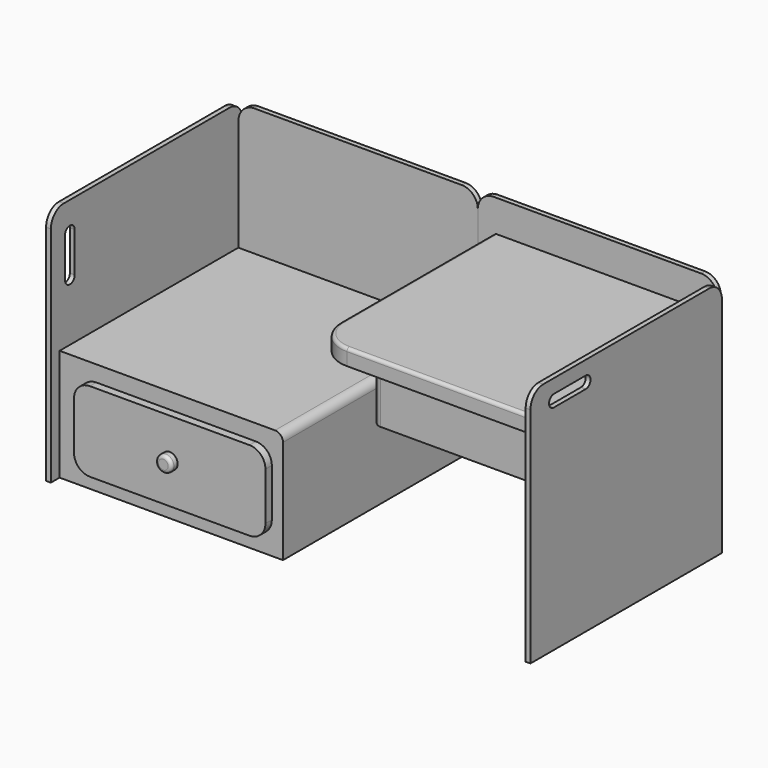
from build123d import *

# Parameters (mm, degrees)
F0_W      = 38.1
F0_H      = 38.1
F2_DEPTH  = 0.762
F1_W      = 38.1
F1_H      = 38.1
F3_DEPTH  = 0.762
F4_W      = 35.56
F4_H      = 35.56
F5_DEPTH  = 17.78
F8_W      = 30.48
F8_H      = 30.48
F9_DEPTH  = 10.16
F7_W      = 35.56
F7_H      = 35.56
F10_DEPTH = 2.54
F11_W     = 30.48
F11_H     = 12.7
F12_DEPTH = 1.27
F13_R     = 1.27
F14_DEPTH = 1.27
F16_R     = 1.27
F17_DEPTH = 2.54
F15_W     = 25.4
F15_H     = 7.62
F18_DEPTH = 1.27
F19_R     = 2.54
F19_2_R   = 2.54
F19_3_R   = 2.54
F20_R     = 5.08
F21_R     = 1.27
F21_2_R   = 1.27
F23_DEPTH = 12.7
F24_DEPTH = 0.762
F26_W     = 38.1
F26_H     = 38.1
F27_DEPTH = 0.762
F29_DEPTH = 12.7
F30_R     = 2.54
F30_2_R   = 2.54
F31_T     = 1.27
F33_DEPTH = 25.4
F34_R     = 0.508
F35_R     = 0.508
F36_R     = 0.508
F38_R     = 1.27


# Not quite as in the source:
# - two fillets or chamfers of one size are made in one step
# - a shell that OpenCascade refuses in one call is made with other operations: the cavity is built on its own and cut out
# - a feature names something its author has since deleted; it is built from what else it names


with BuildPart() as f2:
    # F0 (on Right) → F2 (new body)
    with BuildSketch(Plane.YZ):
        with Locations((-19.05, 19.05)):
            Rectangle(F0_W, F0_H)
    extrude(amount=-F2_DEPTH)

    # F19
    f19_edges = [f2.edges().sort_by_distance(p)[0] for p in [
        (-0.381, -38.1, 38.1),
        (-0.381, 0, 38.1),
    ]]
    fillet(f19_edges, radius=F19_R)

    # F22 (on face) → F23 (cut)
    with BuildSketch(Plane.YZ):
        with BuildLine():
            ThreePointArc((35.283215344, 34.4806989491), (34.330715344, 35.4331989491), (33.378215344, 34.4806989491))
            Line((33.378215344, 34.4806989491), (33.378215344, 28.1306989491))
            ThreePointArc((33.378215344, 28.1306989491), (34.330715344, 27.1781989491), (35.283215344, 28.1306989491))
            Line((35.283215344, 28.1306989491), (35.283215344, 34.4806989491))
        make_face()
    extrude(amount=-F23_DEPTH, mode=Mode.SUBTRACT)

    # F32 (on face) → F33 (cut)
    with BuildSketch(Plane(origin=(-0.762, 0, 0), x_dir=(0, -1, 0), z_dir=(-1, 0, 0))):
        with BuildLine():
            ThreePointArc((35.2714537645, 33.5571871057), (34.3189537645, 34.5096871057), (33.3664537645, 33.5571871057))
            Line((33.3664537645, 33.5571871057), (33.3664537645, 27.2071871057))
            ThreePointArc((33.3664537645, 27.2071871057), (34.3189537645, 26.2546871057), (35.2714537645, 27.2071871057))
            Line((35.2714537645, 27.2071871057), (35.2714537645, 33.5571871057))
        make_face()
    extrude(amount=-F33_DEPTH, mode=Mode.SUBTRACT)


with BuildPart() as f3:
    # F1 (on Front) → F3 (new body)
    with BuildSketch(Plane.XZ):
        with Locations((19.05, 19.05)):
            Rectangle(F1_W, F1_H)
    extrude(amount=F3_DEPTH)

    # F19#2
    f19_2_edges = [f3.edges().sort_by_distance(p)[0] for p in [
        (0, -0.381, 38.1),
        (38.1, -0.381, 38.1),
    ]]
    fillet(f19_2_edges, radius=F19_2_R)


with BuildPart() as f5:
    # F4 (on Top) → F5 (new body)
    with BuildSketch(Plane.XY):
        with Locations((17.78, -18.5785688174)):
            Rectangle(F4_W, F4_H)
    extrude(amount=F5_DEPTH)

    # F21
    f21_edges = [f5.edges().sort_by_distance(p)[0] for p in [
        (35.56, -18.578569, 17.78),
    ]]
    fillet(f21_edges, radius=F21_R)


with BuildPart() as f9:
    # F8 (on offset) → F9 (new body)
    with BuildSketch(Plane.XY.offset(30.48)):
        with Locations((60.96, -16.002)):
            Rectangle(F8_W, F8_H)
    extrude(amount=-F9_DEPTH)

    # F21#2
    f21_2_edges = [f9.edges().sort_by_distance(p)[0] for p in [
        (45.72, -31.242, 25.4),
    ]]
    fillet(f21_2_edges, radius=F21_2_R)

    # F31: shell of thickness 1.27, made by hand


with BuildPart() as f10:
    # F7 (on offset) → F10 (new body)
    with BuildSketch(Plane.XY.offset(30.48)):
        with Locations((58.42, -18.542)):
            Rectangle(F7_W, F7_H)
    extrude(amount=F10_DEPTH)

    # F20
    f20_edges = [f10.edges().sort_by_distance(p)[0] for p in [
        (40.64, -36.322, 31.75),
    ]]
    fillet(f20_edges, radius=F20_R)

    # F34
    f34_edges = [f10.edges().sort_by_distance(p)[0] for p in [
        (40.64, -16.002, 33.02),
    ]]
    fillet(f34_edges, radius=F34_R)


with BuildPart() as f12:
    # F11 (on face) → F12 (new body)
    with BuildSketch(Plane.XZ.offset(36.3585688174)):
        with Locations((18.542, 8.89)):
            Rectangle(F11_W, F11_H)
    extrude(amount=F12_DEPTH)

    # F19#3
    f19_3_edges = [f12.edges().sort_by_distance(p)[0] for p in [
        (3.302, -36.993569, 2.54),
        (33.782, -36.993569, 2.54),
        (33.782, -36.993569, 15.24),
        (3.302, -36.993569, 15.24),
    ]]
    fillet(f19_3_edges, radius=F19_3_R)


with BuildPart() as f14:
    # F13 (on face) → F14 (new body)
    with BuildSketch(Plane.XZ.offset(37.6285688174)):
        with Locations((18.542, 8.89)):
            Circle(F13_R)
    extrude(amount=F14_DEPTH)

    # F35
    f35_edges = [f14.edges().sort_by_distance(p)[0] for p in [
        (17.272, -38.898569, 8.89),
    ]]
    fillet(f35_edges, radius=F35_R)


with BuildPart() as f17:
    # F16 (on face) → F17 (new body)
    with BuildSketch(Plane(origin=(45.72, 0, 0), x_dir=(0, -1, 0), z_dir=(-1, 0, 0))):
        with Locations((16.002, 25.4)):
            Circle(F16_R)
    extrude(amount=F17_DEPTH)

    # F36
    f36_edges = [f17.edges().sort_by_distance(p)[0] for p in [
        (43.18, -14.732, 25.4),
    ]]
    fillet(f36_edges, radius=F36_R)


with BuildPart() as f18:
    # F15 (on face) → F18 (new body)
    with BuildSketch(Plane(origin=(45.72, 0, 0), x_dir=(0, -1, 0), z_dir=(-1, 0, 0))):
        with Locations((16.002, 25.4)):
            Rectangle(F15_W, F15_H)
    extrude(amount=F18_DEPTH)

    # F38
    f38_edges = [f18.edges().sort_by_distance(p)[0] for p in [
        (45.085, -28.702, 21.59),
        (45.085, -28.702, 29.21),
        (45.085, -3.302, 21.59),
        (45.085, -3.302, 29.21),
    ]]
    fillet(f38_edges, radius=F38_R)


with BuildPart() as f24:
    # F1 (on Front) → F24 (new body)
    with BuildSketch(Plane.XZ):
        with Locations((57.15, 19.05)):
            Rectangle(F1_W, F1_H)
    extrude(amount=F24_DEPTH)

    # F30
    f30_edges = [f24.edges().sort_by_distance(p)[0] for p in [
        (76.2, -0.381, 38.1),
        (38.1, -0.381, 38.1),
    ]]
    fillet(f30_edges, radius=F30_R)


with BuildPart() as f27:
    # F26 (on offset) → F27 (new body)
    with BuildSketch(Plane.YZ.offset(76.2)):
        with Locations((-19.812, 19.05)):
            Rectangle(F26_W, F26_H)
    extrude(amount=F27_DEPTH)

    # F28 (on face) → F29 (cut)
    with BuildSketch(Plane.YZ.offset(76.962)):
        with BuildLine():
            Line((-27.8631728142, 35.8923991907), (-34.2131728142, 35.8923991907))
            ThreePointArc((-34.2131728142, 35.8923991907), (-35.1656728142, 34.9398991907), (-34.2131728142, 33.9873991907))
            Line((-34.2131728142, 33.9873991907), (-27.8631728142, 33.9873991907))
            ThreePointArc((-27.8631728142, 33.9873991907), (-26.9106728142, 34.9398991907), (-27.8631728142, 35.8923991907))
        make_face()
    extrude(amount=-F29_DEPTH, mode=Mode.SUBTRACT)

    # F30#2
    f30_2_edges = [f27.edges().sort_by_distance(p)[0] for p in [
        (76.581, -0.762, 38.1),
        (76.581, -38.862, 38.1),
    ]]
    fillet(f30_2_edges, radius=F30_2_R)


with BuildPart() as f31_core1:
    # F31_t2: copy of F9
    add(f9.part)

    # the walls: a layer under each face that stays
    f31_faces = [f31_core1.faces().sort_by_distance(p)[0] for p in [
        (45.72, -15.367, 25.4),
        (60.96, -16.002, 30.48),
        (60.96, -0.762, 25.4),
        (61.595, -31.242, 25.4),
        (76.2, -16.002, 25.4),
    ]]
    thicken(f31_faces, amount=-F31_T, mode=Mode.SUBTRACT)


with BuildPart() as f9_1:
    add(f9.part)

    # what is left inside the walls is the cavity
    f31_cavity = [f31_core1.part.solids().sort_by_distance(p)[0] for p in [
        (60.96, -20.658667, 20.3327),
    ]]
    add(f31_cavity, mode=Mode.SUBTRACT)


solid = Compound([f2.part, f3.part, f5.part, f10.part, f12.part, f14.part, f17.part, f18.part, f24.part, f27.part, f9_1.part])
